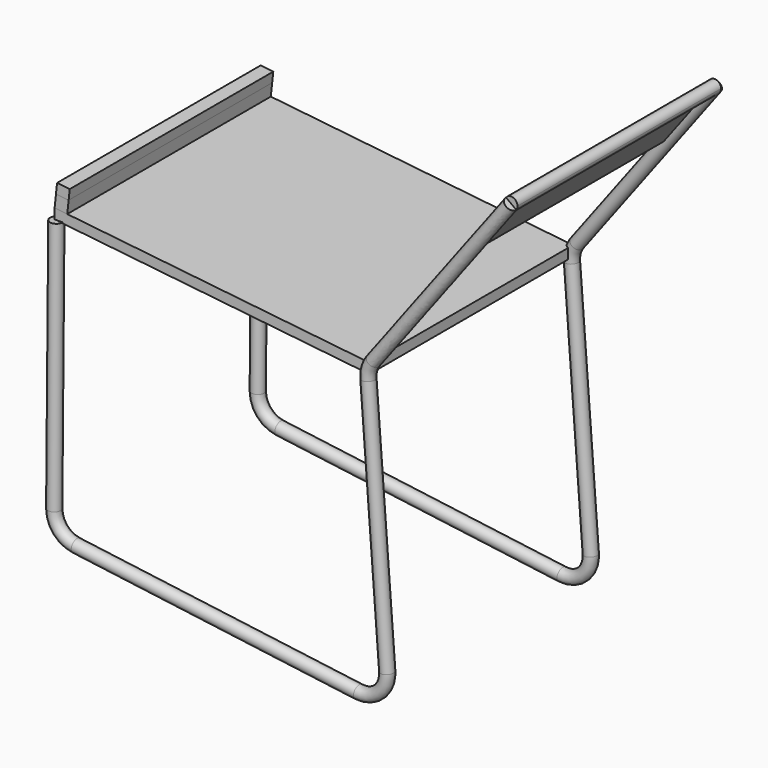
from build123d import *

# Parameters (mm, degrees)
F4_R      = 6.35
F6_R      = 6.35
F8_DEPTH  = 254
F10_W     = 254
F10_H     = 10.16
F14_DEPTH = 254
F15_W     = 12.7
F15_H     = 254
F16_DEPTH = 12.7
F17_W     = 12.7
F17_H     = 254
F18_DEPTH = 10.16


with BuildPart() as f5:
    # F5: sweep along a path in F1
    with BuildLine(Plane.XZ) as f5_path:
        Line((-61.7453475377, 208.0074561836), (-63.8906607053, -45.9834838741))
        ThreePointArc((-63.8906607053, -45.9834838741), (-57.6518689096, -62.872631205), (-41.7858294707, -71.3834838741))
        Line((-41.7858294707, -71.3834838741), (239.9254137755, -108.2313532754))
        ThreePointArc((239.9254137755, -108.2313532754), (260.675596222, -101.4971953394), (268.5489681957, -81.1519509704))
        Line((268.5489681957, -81.1519509704), (249.7536663039, 170.2146638692))
        ThreePointArc((249.7536663039, 170.2146638692), (250.7094665663, 179.2565284944), (254.7884130124, 187.38247865))
        Line((254.7884130124, 187.38247865), (392.253343443, 370.0333831145))
    # F4 (on offset) → F5 (sweep)
    with BuildSketch(Plane.XY.offset(208.007458)):
        with Locations((-61.7453475377, 0)):
            Circle(F4_R)
    sweep(path=f5_path.line)


with BuildPart() as f7:
    # F7: sweep along a path in F2
    with BuildLine(Plane.XZ.offset(254)) as f7_path:
        Line((-61.7453475377, 208.0074561836), (-63.8906607053, -45.9834838741))
        ThreePointArc((-63.8906607053, -45.9834838741), (-57.6518689096, -62.872631205), (-41.7858294707, -71.3834838741))
        Line((-41.7858294707, -71.3834838741), (239.9254137755, -108.2313532754))
        ThreePointArc((239.9254137755, -108.2313532754), (260.675596222, -101.4971953394), (268.5489681957, -81.1519509704))
        Line((268.5489681957, -81.1519509704), (249.7536663039, 170.2146638692))
        ThreePointArc((249.7536663039, 170.2146638692), (250.7094665663, 179.2565284944), (254.7884130124, 187.38247865))
        Line((254.7884130124, 187.38247865), (392.253343443, 370.0333831145))
    # F6 (on offset) → F7 (sweep)
    with BuildSketch(Plane.XY.offset(208.007458)):
        with Locations((-61.7453475377, -254)):
            Circle(F6_R)
    sweep(path=f7_path.line)

    # F2 (on offset) → F8 (join)
    with BuildSketch(Plane.XZ.offset(254)):
        with BuildLine():
            ThreePointArc((388.4348731532, 364.9597468793), (395.0884107843, 364.3514034269), (398.603343443, 370.0333831145))
            ThreePointArc((398.603343443, 370.0333831145), (389.4182761016, 375.715362802), (388.4348731532, 364.9597468793))
        make_face()
    extrude(amount=-F8_DEPTH)

    # F13 (on face) → F14 (join)
    with BuildSketch(Plane.XZ.offset(254)):
        Polygon((392.253343443, 370.0333831145), (385.903343443, 370.0333831145), (340.0816999661, 309.149748293), (346.4316999661, 309.149748293), align=None)
    extrude(amount=-F14_DEPTH)


with BuildPart() as f12:
    # F12: sweep along a path in F11
    with BuildLine(Plane.XZ) as f12_path:
        Line((-63.5, 213.0874561836), (250.7094665663, 179.2565284944))
    # F10 (on offset) → F12 (sweep)
    with BuildSketch(Plane.YZ.offset(-63.5)):
        with Locations((-127, 213.0874561836)):
            Rectangle(F10_W, F10_H)
    sweep(path=f12_path.line)


with BuildPart() as f16:
    # F15 (on face) → F16 (new body)
    with BuildSketch(Plane(origin=(22.4931822163, 0, 208.9085717804), x_dir=(0.9942535031, 0, -0.107051257), z_dir=(0.107051257, 0, 0.9942535031))):
        with Locations((-80.1401978729, -127)):
            Rectangle(F15_W, F15_H)
    extrude(amount=F16_DEPTH)


with BuildPart() as f18:
    # F17 (on face) → F18 (new body)
    with BuildSketch(Plane(origin=(23.8527331806, 0, 221.5355912694), x_dir=(0.9942535031, 0, -0.107051257), z_dir=(0.107051257, 0, 0.9942535031))):
        with Locations((-80.1401978729, -127)):
            Rectangle(F17_W, F17_H)
    extrude(amount=F18_DEPTH)


solid = Compound([f5.part, f7.part, f12.part, f16.part, f18.part])
